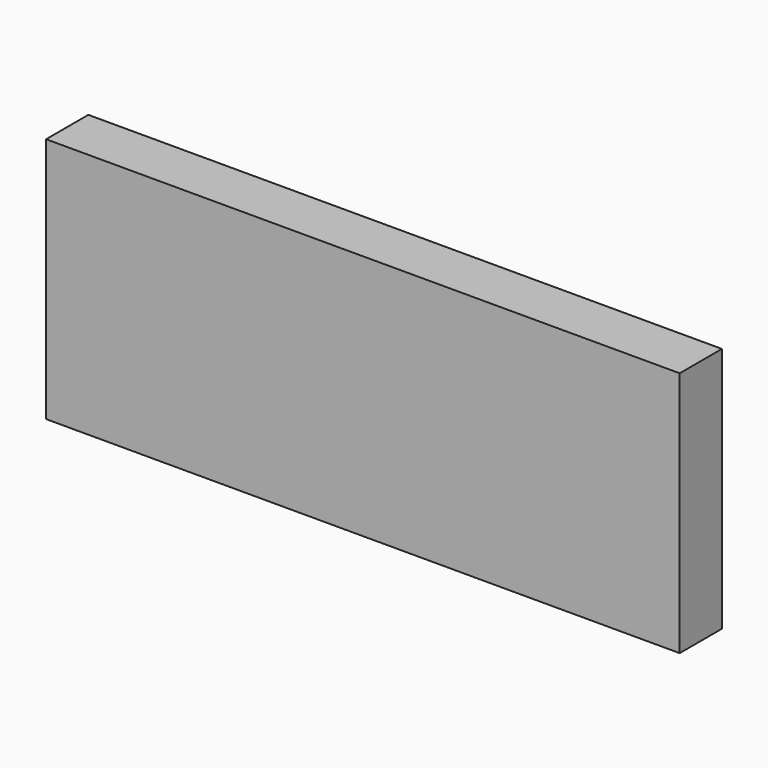
from build123d import *

# Parameters (mm, degrees)
F1_W     = 19.05
F1_H     = 88.9
F2_DEPTH = 228.6


# Not quite as in the source:
# - a variable given as a bare number and used for a length is read in inches; the dataset says mm whatever the document's units were


with BuildPart() as f2:
    # F1 (on Right) → F2 (new body)
    with BuildSketch(Plane.YZ):
        with Locations((9.525, 44.45)):
            Rectangle(F1_W, F1_H)
    extrude(amount=-F2_DEPTH)


solid = f2.part
